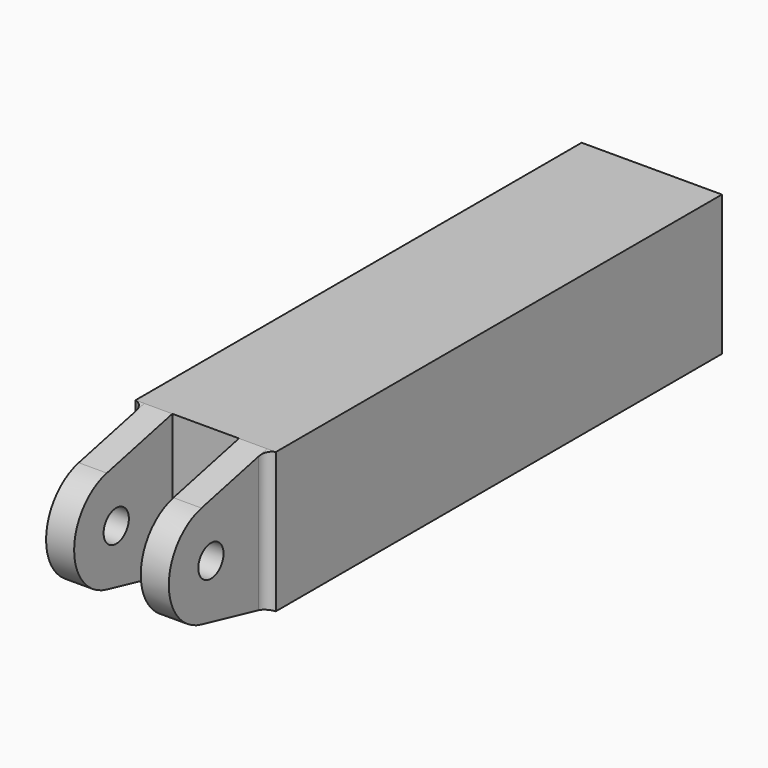
from build123d import *

# Parameters (mm, degrees)
F0_W         = 160
F0_H         = 40
F1_DEPTH     = 20
F2_W         = 34
F2_H         = 34
F3_DEPTH     = 25
F4_R         = 4.5
F5_DEPTH     = 17.5
F7_DEPTH     = 25
F8_T4_DEPTH  = 54.7901994578
F8_T10_DEPTH = 54.7901994578
F9_SIZE      = 1


# Not quite as in the source:
# - a fillet or chamfer that OpenCascade refuses, or shapes differently, is made with other operations: its cross-section is extruded or revolved along the edge and cut away or added


with BuildPart() as f1:
    # F0 (on Right) → F1 (new body, symmetric)
    with BuildSketch(Plane.YZ):
        Rectangle(F0_W, F0_H)
    extrude(amount=F1_DEPTH, both=True)

    # F2 (on face) → F3 (cut)
    with BuildSketch(Plane(origin=(0, 80, 0), x_dir=(-1, 0, 0), z_dir=(0, 1, 0))):
        Rectangle(F2_W, F2_H)
    extrude(amount=-F3_DEPTH, mode=Mode.SUBTRACT)

    # F4 (on Right) → F5 (join, symmetric)
    with BuildSketch(Plane.YZ):
        with BuildLine():
            Line((-80, 20), (-103.3671841062, 14.6171841062))
            ThreePointArc((-103.3671841062, 14.6171841062), (-115, 0), (-103.3671841062, -14.6171841062))
            Line((-103.3671841062, -14.6171841062), (-80, -20))
            Line((-80, -20), (-80, 0))
            Line((-80, 0), (-80, 20))
        make_face()
        with Locations((-100, 0)):
            Circle(F4_R, mode=Mode.SUBTRACT)
    extrude(amount=F5_DEPTH, both=True)

    # F6 (on Top) → F7 (cut, symmetric)
    with BuildSketch(Plane.XY):
        Polygon((-9.5, -115), (0, -115), (9.5, -115), (9.5, -80), (-9.5, -80), align=None)
    extrude(amount=F7_DEPTH, both=True, mode=Mode.SUBTRACT)

    # F8: fillet of radius 3 on 2 edges, made by hand


with BuildPart() as f8_tool2:
    # F8_s3 → F8_t4 (new body)
    with BuildSketch(Plane.XY.offset(-27.3950997289)):
        with BuildLine():
            ThreePointArc((-17.5, -82.9580398916), (-18.2087121525, -81.0215482184), (-20, -80))
            Line((-20, -80), (-17.5, -80))
            Line((-17.5, -80), (-17.5, -82.9580398916))
        make_face()
    extrude(amount=F8_T4_DEPTH)

    split(bisect_by=Plane(origin=(0, -8.4062635752, 36.4921841062), x_dir=(1, 0, 0), z_dir=(0, 0.2244789404, -0.9744789404)), keep=Keep.TOP)

    split(bisect_by=Plane(origin=(0, -8.4062635752, -36.4921841062), x_dir=(1, 0, 0), z_dir=(0, 0.2244789404, 0.9744789404)), keep=Keep.TOP)


with BuildPart() as f1_1:
    add(f1.part)

    # F8_t1: union F8_tool2
    add(f8_tool2.part)


with BuildPart() as f8_tool8:
    # F8_s9 → F8_t10 (new body)
    with BuildSketch(Plane.XY.offset(27.3950997289)):
        with BuildLine():
            ThreePointArc((20, -80), (18.2087121525, -81.0215482184), (17.5, -82.9580398916))
            Line((17.5, -82.9580398916), (17.5, -80))
            Line((17.5, -80), (20, -80))
        make_face()
    extrude(amount=-F8_T10_DEPTH)

    split(bisect_by=Plane(origin=(0, -8.4062635752, -36.4921841062), x_dir=(1, 0, 0), z_dir=(0, 0.2244789404, 0.9744789404)), keep=Keep.TOP)

    split(bisect_by=Plane(origin=(0, -8.4062635752, 36.4921841062), x_dir=(1, 0, 0), z_dir=(0, 0.2244789404, -0.9744789404)), keep=Keep.TOP)


with BuildPart() as f1_2:
    add(f1_1.part)

    # F8_t7: union F8_tool8
    add(f8_tool8.part)

    # F9
    f9_edges = [f1_2.edges().sort_by_distance(p)[0] for p in [
        (0, 80, 20),
        (-20, 80, 0),
        (0, 80, -20),
        (20, 80, 0),
    ]]
    chamfer(f9_edges, length=F9_SIZE)


solid = f1_2.part
